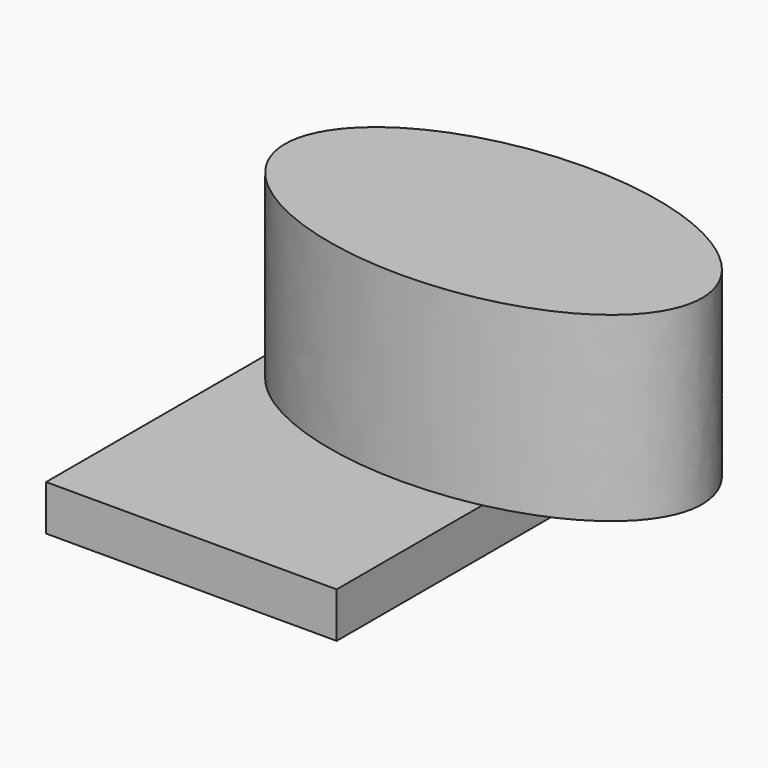
from build123d import *

# Parameters (mm, degrees)
F0_W     = 40.64
F0_H     = 40.64
F1_DEPTH = 6.35
F2_W     = 35.56
F2_H     = 35.56
F3_DEPTH = 1.27
F5_DEPTH = 25.4


# Not quite as in the source:
# - a feature names something its author has since deleted; it is built from what else it names


with BuildPart() as f1:
    # F0 (on Top) → F1 (new body)
    with BuildSketch(Plane.XY):
        Rectangle(F0_W, F0_H)
    extrude(amount=F1_DEPTH)

    # F2 (on Top) → F3 (join)
    with BuildSketch(Plane.XY):
        Rectangle(F2_W, F2_H)
    extrude(amount=F3_DEPTH)

    # F4 (on face) → F5 (join)
    with BuildSketch(Plane.XY.offset(6.35)):
        with BuildLine():
            add(Edge.make_bspline(
                [(9.7486972809, 4.0494650602), (60.2697605827, 4.0494650602), (35.0092289318, 28.4552674699), (9.7486972809, 52.8610698795), (-15.51183437, 28.4552674699), (-40.7723660209, 4.0494650602), (9.7486972809, 4.0494650602)],
                knots=[4.7123889804, 4.7123889804, 4.7123889804, 6.8067840828, 6.8067840828, 8.9011791852, 8.9011791852, 10.9955742876, 10.9955742876, 10.9955742876], degree=2, weights=[1, 0.5, 1, 0.5, 1, 0.5, 1]))
        make_face()
    extrude(amount=F5_DEPTH)


solid = f1.part
